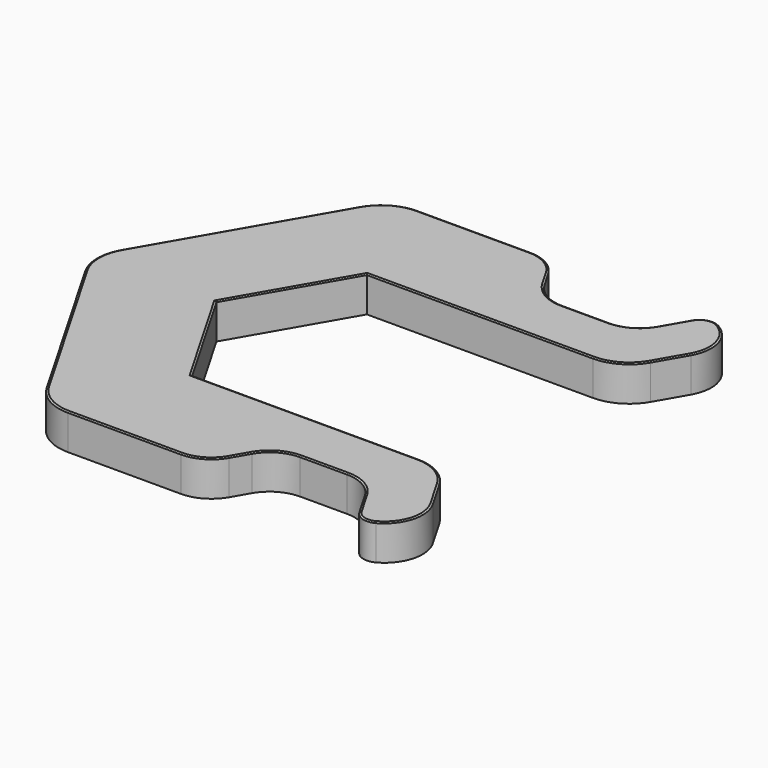
from build123d import *

# Parameters (mm, degrees)
F1_DEPTH      = 4
F2_R          = 5
F3_T1_DEPTH   = 4
F3_T3_DEPTH   = 4
F3_T5_DEPTH   = 40.2941740367
F3_T7_DEPTH   = 16.124355653
F4_R          = 1.75
F6_R          = 5
F7_T1_DEPTH   = 21.9393102292
F7_T3_DEPTH   = 21.9393102292
F7_T5_DEPTH   = 12.4011904446
F7_T7_DEPTH   = 2.0784609691
F7_T9_DEPTH   = 2.0784609691
F7_T11_DEPTH  = 5.1502577388
F7_T13_DEPTH  = 3.1580886503
F7_T15_DEPTH  = 3.1580886503
F7_T17_DEPTH  = 3.7108203073
F7_T19_DEPTH  = 3.7108203073
F7_T22_ANGLE  = 60
F7_T24_ANGLE  = 60
F7_T26_ANGLE  = 60
F7_T28_ANGLE  = 60.000000004
F7_T30_ANGLE  = 60.000000004
F7_T32_ANGLE  = 60.0000000003
F7_T34_ANGLE  = 60.0000000003
F7_T36_ANGLE  = 60.0000000003
F7_T38_ANGLE  = 60.0000000003
F7_T40_ANGLE  = 88.8306171943
F7_T42_ANGLE  = 91.1693828062
F7_T44_ANGLE  = 88.8306171943
F7_T46_ANGLE  = 91.1693828062
F7_T48_ANGLE  = 60
F7_T52_DEPTH  = 25.3440273499
F7_T55_ANGLE  = 60
F7_T59_DEPTH  = 14.8923380101
F7_T65_DEPTH  = 25.3440273499
F7_T70_DEPTH  = 14.8923380101
F7_T76_DEPTH  = 14.8923380101
F7_T82_DEPTH  = 14.8923380101
F7_T86_ANGLE  = 60
F7_T88_ANGLE  = 60
F7_T90_ANGLE  = 60
F7_T92_ANGLE  = 60.000000004
F7_T94_ANGLE  = 60.000000004
F7_T96_ANGLE  = 60.0000000003
F7_T98_ANGLE  = 60.0000000003
F7_T100_ANGLE = 60.0000000003
F7_T102_ANGLE = 60.0000000003
F7_T104_ANGLE = 88.8306171943
F7_T106_ANGLE = 91.1693828062
F7_T108_ANGLE = 88.8306171943
F7_T110_ANGLE = 91.1693828062
F7_T112_ANGLE = 60
F7_T116_DEPTH = 25.3440273499
F7_T119_ANGLE = 60
F7_T123_DEPTH = 25.3440273499
F7_T129_DEPTH = 25.3440273499
F7_T133_DEPTH = 14.8923380101
F7_T140_DEPTH = 14.8923380101
F7_T144_DEPTH = 14.8923380101
F7_T151_DEPTH = 25.3440273499
F7_T155_DEPTH = 14.8923380101
F7_T162_DEPTH = 25.3440273499
F7_T166_DEPTH = 14.8923380101
F7_T173_DEPTH = 14.8923380101
F7_T177_DEPTH = 14.8923380101
F7_T184_DEPTH = 25.3440273499
F7_T188_DEPTH = 14.8923380101


# Not quite as in the source:
# - a fillet or chamfer that OpenCascade refuses, or shapes differently, is made with other operations: its cross-section is extruded or revolved along the edge and cut away or added


with BuildPart() as f1:
    # F0 (on Top) → F1 (new body)
    with BuildSketch(Plane.XY):
        Polygon((20.7846096908, -12), (6.9282032303, -12), (-6.9282032303, -12), (-13.8564064606, 0), (-27.7128129211, 0), (-13.8564064606, -24), (3.8564064606, -24), (7.3205080757, -18), (17.3205080757, -18), align=None)
        Polygon((27.7128129211, -24), (20.7846096908, -12), (17.3205080757, -18), (20.7846096908, -24), align=None)
    extrude(amount=F1_DEPTH)

    # F2
    f2_edges = [f1.edges().sort_by_distance(p)[0] for p in [
        (-13.856406, -24, 2),
        (20.78461, -12, 2),
    ]]
    fillet(f2_edges, radius=F2_R)

    # F3: fillet of radius 4.2 on 4 edges, made by hand

    # F3_s2 → F3_t1 (join)
    with BuildSketch(Plane.XY):
        with BuildLine():
            ThreePointArc((18.532943641, -20.1), (16.9956369451, -18.5626933041), (14.8956369451, -18))
            Line((14.8956369451, -18), (17.3205080757, -18))
            Line((17.3205080757, -18), (18.532943641, -20.1))
        make_face()
    extrude(amount=F3_T1_DEPTH)

    # F3_s4 → F3_t3 (join)
    with BuildSketch(Plane.XY):
        with BuildLine():
            ThreePointArc((9.7453792063, -18), (7.6453792063, -18.5626933041), (6.1080725104, -20.1))
            Line((6.1080725104, -20.1), (7.3205080757, -18))
            Line((7.3205080757, -18), (9.7453792063, -18))
        make_face()
    extrude(amount=F3_T3_DEPTH)

    # F3_s6 → F3_t5 (cut)
    with BuildSketch(Plane.XY.offset(-18.1470870184)):
        with BuildLine():
            ThreePointArc((20.7846096908, -24), (24.165134966, -21.7652526687), (24.0833955174, -17.713664655))
            Line((24.0833955174, -17.713664655), (27.7128129211, -24))
            Line((27.7128129211, -24), (20.7846096908, -24))
        make_face()
    extrude(amount=F3_T5_DEPTH, mode=Mode.SUBTRACT)

    # F3_s8 → F3_t7 (cut)
    with BuildSketch(Plane.XY.offset(-6.0621778265)):
        with BuildLine():
            ThreePointArc((5.0688420258, -21.9), (3.53153533, -23.4373066959), (1.43153533, -24))
            Line((1.43153533, -24), (3.8564064606, -24))
            Line((3.8564064606, -24), (5.0688420258, -21.9))
        make_face()
    extrude(amount=F3_T7_DEPTH, mode=Mode.SUBTRACT)

    # F4
    f4_edges = [f1.edges().sort_by_distance(p)[0] for p in [
        (20.78461, -24, 2),
    ]]
    fillet(f4_edges, radius=F4_R)

    # F5: F1 across face


with BuildPart() as f1_1:
    add(f1.part)
    add(f1.part.mirror(Plane(origin=(-20.7846096908, 0, 2), x_dir=(-1, 0, 0), z_dir=(0, 1, 0))))

    # F6
    f6_edges = [f1_1.edges().sort_by_distance(p)[0] for p in [
        (-27.712813, 0, 2),
    ]]
    fillet(f6_edges, radius=F6_R)

    # F7: chamfer of 0.2 x 0.1 on 62 edges, made by hand

    # F7_s2 → F7_t1 (cut)
    with BuildSketch(Plane(origin=(-5.4848275573, -9.5, 0), x_dir=(0, 0, 1), z_dir=(0.5, 0.8660254038, 0))):
        Polygon((3.9, -24), (4, -23.8), (4, -24), align=None)
        Polygon((0, -23.8), (0.1, -24), (0, -24), align=None)
    extrude(amount=F7_T1_DEPTH, mode=Mode.SUBTRACT)

    # F7_s4 → F7_t3 (cut)
    with BuildSketch(Plane(origin=(-5.4848275573, 9.5, 0), x_dir=(0, 0, 1), z_dir=(0.5, -0.8660254038, 0))):
        Polygon((3.9, 24), (4, 23.8), (4, 24), align=None)
        Polygon((0, 23.8), (0.1, 24), (0, 24), align=None)
    extrude(amount=F7_T3_DEPTH, mode=Mode.SUBTRACT)

    # F7_s6 → F7_t5 (cut)
    with BuildSketch(Plane.YZ.offset(-10.9696551146)):
        Polygon((24, 3.9), (23.8, 4), (24, 4), align=None)
        Polygon((-24, 3.9), (-23.8, 4), (-24, 4), align=None)
        Polygon((-23.8, 0), (-24, 0.1), (-24, 0), align=None)
        Polygon((23.8, 0), (24, 0.1), (24, 0), align=None)
    extrude(amount=F7_T5_DEPTH, mode=Mode.SUBTRACT)

    # F7_s8 → F7_t7 (cut)
    with BuildSketch(Plane(origin=(-8.215767665, 14.2301270189, 0), x_dir=(0, 0, 1), z_dir=(0.5, -0.8660254038, 0))):
        Polygon((3.9, -15.3397459622), (4, -15.1397459622), (4, -15.3397459622), align=None)
        Polygon((0, -15.1397459622), (0.1, -15.3397459622), (0, -15.3397459622), align=None)
    extrude(amount=F7_T7_DEPTH, mode=Mode.SUBTRACT)

    # F7_s10 → F7_t9 (cut)
    with BuildSketch(Plane(origin=(-8.215767665, -14.2301270189, 0), x_dir=(0, 0, 1), z_dir=(0.5, 0.8660254038, 0))):
        Polygon((3.9, 15.3397459622), (4, 15.1397459622), (4, 15.3397459622), align=None)
        Polygon((0, 15.1397459622), (0.1, 15.3397459622), (0, 15.3397459622), align=None)
    extrude(amount=F7_T9_DEPTH, mode=Mode.SUBTRACT)

    # F7_s12 → F7_t11 (cut)
    with BuildSketch(Plane.YZ.offset(9.7453792063)):
        Polygon((18, 3.9), (17.8, 4), (18, 4), align=None)
        Polygon((-18, 3.9), (-17.8, 4), (-18, 4), align=None)
        Polygon((17.8, 0), (18, 0.1), (18, 0), align=None)
        Polygon((-17.8, 0), (-18, 0.1), (-18, 0), align=None)
    extrude(amount=F7_T11_DEPTH, mode=Mode.SUBTRACT)

    # F7_s14 → F7_t13 (cut)
    with BuildSketch(Plane(origin=(13.3367912183, 23.1, 0), x_dir=(0, 0, 1), z_dir=(0.5, 0.8660254038, 0))):
        Polygon((3.9, 6), (4, 6.2), (4, 6), align=None)
        Polygon((0, 6.2), (0.1, 6), (0, 6), align=None)
    extrude(amount=F7_T13_DEPTH, mode=Mode.SUBTRACT)

    # F7_s16 → F7_t15 (cut)
    with BuildSketch(Plane(origin=(13.3367912183, -23.1, 0), x_dir=(0, 0, 1), z_dir=(0.5, -0.8660254038, 0))):
        Polygon((3.9, -6), (4, -6.2), (4, -6), align=None)
        Polygon((0, -6.2), (0.1, -6), (0, -6), align=None)
    extrude(amount=F7_T15_DEPTH, mode=Mode.SUBTRACT)

    # F7_s18 → F7_t17 (cut)
    with BuildSketch(Plane(origin=(13.691090672, 23.713664655, 0), x_dir=(0, 0, 1), z_dir=(-0.5, -0.8660254038, 0))):
        Polygon((3.9, -12), (4, -11.8), (4, -12), align=None)
        Polygon((0, -11.8), (0.1, -12), (0, -12), align=None)
    extrude(amount=F7_T17_DEPTH, mode=Mode.SUBTRACT)

    # F7_s20 → F7_t19 (cut)
    with BuildSketch(Plane(origin=(13.691090672, -23.713664655, 0), x_dir=(0, 0, 1), z_dir=(-0.5, 0.8660254038, 0))):
        Polygon((3.9, 12), (4, 11.8), (4, 12), align=None)
        Polygon((0, 11.8), (0.1, 12), (0, 12), align=None)
    extrude(amount=F7_T19_DEPTH, mode=Mode.SUBTRACT)

    # F7_s21 → F7_t22 (revolve, cut)
    with BuildSketch(Plane(origin=(-5.4848275573, 9.5, 0), x_dir=(0, 0, 1), z_dir=(0.5, -0.8660254038, 0))):
        Polygon((3.9, 24), (4, 23.8), (4, 24), align=None)
    revolve(axis=Axis((-21.9393102292, 0, 4), (0, 0, -1)), revolution_arc=F7_T22_ANGLE, mode=Mode.SUBTRACT)

    # F7_s23 → F7_t24 (revolve, cut)
    with BuildSketch(Plane(origin=(5.4848275573, 9.5, 0), x_dir=(0, 0, 1), z_dir=(-0.5, -0.8660254038, 0))):
        Polygon((3.9, 24), (4, 23.8), (4, 24), align=None)
    revolve(axis=Axis((-10.9696551146, 19, 4), (0, 0, -1)), revolution_arc=F7_T24_ANGLE, mode=Mode.SUBTRACT)

    # F7_s25 → F7_t26 (revolve, cut)
    with BuildSketch(Plane(origin=(5.4848275573, -9.5, 0), x_dir=(0, 0, 1), z_dir=(-0.5, 0.8660254038, 0))):
        Polygon((3.9, -24), (4, -23.8), (4, -24), align=None)
    revolve(axis=Axis((-10.9696551146, -19, 4), (0, 0, 1)), revolution_arc=F7_T26_ANGLE, mode=Mode.SUBTRACT)

    # F7_s27 → F7_t28 (revolve, cut)
    with BuildSketch(Plane(origin=(-8.2157676647, 14.2301270199, 0), x_dir=(0, 0, 1), z_dir=(0.5, -0.8660254038, 0))):
        Polygon((3.9, -15.3397459614), (4, -15.1397459614), (4, -15.3397459614), align=None)
    revolve(axis=Axis((1.4315353301, 19.8000000003, 4), (0, 0, 1)), revolution_arc=F7_T28_ANGLE, mode=Mode.SUBTRACT)

    # F7_s29 → F7_t30 (revolve, cut)
    with BuildSketch(Plane(origin=(-8.2157676647, -14.2301270199, 0), x_dir=(0, 0, 1), z_dir=(0.5, 0.8660254038, 0))):
        Polygon((3.9, 15.3397459614), (4, 15.1397459614), (4, 15.3397459614), align=None)
    revolve(axis=Axis((1.4315353301, -19.8000000003, 4), (0, 0, -1)), revolution_arc=F7_T30_ANGLE, mode=Mode.SUBTRACT)

    # F7_s31 → F7_t32 (revolve, cut)
    with BuildSketch(Plane.YZ.offset(9.7453792063)):
        Polygon((18, 3.9), (17.8, 4), (18, 4), align=None)
    revolve(axis=Axis((9.7453792063, 22.2, 4), (0, 0, -1)), revolution_arc=F7_T32_ANGLE, mode=Mode.SUBTRACT)

    # F7_s33 → F7_t34 (revolve, cut)
    with BuildSketch(Plane.YZ.offset(9.7453792063)):
        Polygon((-18, 3.9), (-17.8, 4), (-18, 4), align=None)
    revolve(axis=Axis((9.7453792063, -22.2, 4), (0, 0, 1)), revolution_arc=F7_T34_ANGLE, mode=Mode.SUBTRACT)

    # F7_s35 → F7_t36 (revolve, cut)
    with BuildSketch(Plane(origin=(13.3367912182, 23.1, 0), x_dir=(0, 0, 1), z_dir=(0.5, 0.8660254038, 0))):
        Polygon((3.9, 6.0000000001), (4, 6.2000000001), (4, 6.0000000001), align=None)
    revolve(axis=Axis((14.8956369451, 22.2, 4), (0, 0, -1)), revolution_arc=F7_T36_ANGLE, mode=Mode.SUBTRACT)

    # F7_s37 → F7_t38 (revolve, cut)
    with BuildSketch(Plane(origin=(13.3367912182, -23.1, 0), x_dir=(0, 0, 1), z_dir=(0.5, -0.8660254038, 0))):
        Polygon((3.9, -6.0000000001), (4, -6.2000000001), (4, -6.0000000001), align=None)
    revolve(axis=Axis((14.8956369451, -22.2, 4), (0, 0, 1)), revolution_arc=F7_T38_ANGLE, mode=Mode.SUBTRACT)

    # F7_s39 → F7_t40 (revolve, cut)
    with BuildSketch(Plane(origin=(7.3213137927, -4.0300225261, 0), x_dir=(0, 0, 1), z_dir=(0.8760491198, -0.482221878, 0))):
        Polygon((3.9, -31.4172948315), (4, -31.2172948315), (4, -31.4172948315), align=None)
    revolve(axis=Axis((21.6275324227, 21.9599849985, 4), (0, 0, 1)), revolution_arc=F7_T40_ANGLE, mode=Mode.SUBTRACT)

    # F7_s41 → F7_t42 (revolve, cut)
    with BuildSketch(Plane(origin=(13.6910906723, 23.7136646549, 0), x_dir=(0, 0, 1), z_dir=(-0.5, -0.8660254038, 0))):
        Polygon((3.9, -11.9999999997), (4, -11.7999999997), (4, -11.9999999997), align=None)
    revolve(axis=Axis((20.4460888216, 19.813664655, 4), (0, 0, 1)), revolution_arc=F7_T42_ANGLE, mode=Mode.SUBTRACT)

    # F7_s43 → F7_t44 (revolve, cut)
    with BuildSketch(Plane(origin=(7.3213137927, 4.0300225261, 0), x_dir=(0, 0, 1), z_dir=(0.8760491198, 0.482221878, 0))):
        Polygon((3.9, 31.4172948315), (4, 31.2172948315), (4, 31.4172948315), align=None)
    revolve(axis=Axis((21.6275324227, -21.9599849985, 4), (0, 0, -1)), revolution_arc=F7_T44_ANGLE, mode=Mode.SUBTRACT)

    # F7_s45 → F7_t46 (revolve, cut)
    with BuildSketch(Plane(origin=(13.6910906723, -23.7136646549, 0), x_dir=(0, 0, 1), z_dir=(-0.5, 0.8660254038, 0))):
        Polygon((3.9, 11.9999999997), (4, 11.7999999997), (4, 11.9999999997), align=None)
    revolve(axis=Axis((20.4460888216, -19.813664655, 4), (0, 0, -1)), revolution_arc=F7_T46_ANGLE, mode=Mode.SUBTRACT)

    # F7_s47 → F7_t48 (revolve, cut)
    with BuildSketch(Plane.YZ.offset(17.8978583449)):
        Polygon((12, 3.9), (12.2, 4), (12, 4), align=None)
    revolve(axis=Axis((17.8978583449, 17, 4), (0, 0, 1)), revolution_arc=F7_T48_ANGLE, mode=Mode.SUBTRACT)


with BuildPart() as f7_tool50:
    # F7_s51 → F7_t52 (new body)
    with BuildSketch(Plane.YZ.offset(17.8978583449)):
        Polygon((12, 3.9), (12.2, 4), (12, 4), align=None)
    extrude(amount=-F7_T52_DEPTH)

    split(bisect_by=Plane(origin=(-10.3923048454, 6, 0), x_dir=(0, 0, 1), z_dir=(0.8660254038, -0.5, 0)), keep=Keep.TOP)


with BuildPart() as f1_2:
    add(f1_1.part)

    # F7_t49: cut F7_tool50
    add(f7_tool50.part, mode=Mode.SUBTRACT)

    # F7_s54 → F7_t55 (revolve, cut)
    with BuildSketch(Plane.YZ.offset(17.8978583449)):
        Polygon((-12, 3.9), (-12.2, 4), (-12, 4), align=None)
    revolve(axis=Axis((17.8978583449, -17, 4), (0, 0, -1)), revolution_arc=F7_T55_ANGLE, mode=Mode.SUBTRACT)


with BuildPart() as f7_tool57:
    # F7_s58 → F7_t59 (new body)
    with BuildSketch(Plane(origin=(3.7230845025, 6.4485715192, 0), x_dir=(0, 0, 1), z_dir=(-0.5, -0.8660254038, 0))):
        Polygon((3.9, 12), (4, 12.2), (4, 12), align=None)
    extrude(amount=F7_T59_DEPTH)

    split(bisect_by=Plane.XZ.offset(-12), keep=Keep.TOP)

    split(bisect_by=Plane(origin=(-10.3923048454, -6, 0), x_dir=(0, 0, 1), z_dir=(0.8660254038, 0.5, 0)), keep=Keep.TOP)


with BuildPart() as f1_3:
    add(f1_2.part)

    # F7_t56: cut F7_tool57
    add(f7_tool57.part, mode=Mode.SUBTRACT)


with BuildPart() as f7_tool63:
    # F7_s64 → F7_t65 (new body)
    with BuildSketch(Plane.YZ.offset(17.8978583449)):
        Polygon((-12, 3.9), (-12.2, 4), (-12, 4), align=None)
    extrude(amount=-F7_T65_DEPTH)

    split(bisect_by=Plane(origin=(-10.3923048454, -6, 0), x_dir=(0, 0, 1), z_dir=(0.8660254038, 0.5, 0)), keep=Keep.TOP)


with BuildPart() as f1_4:
    add(f1_3.part)

    # F7_t62: cut F7_tool63
    add(f7_tool63.part, mode=Mode.SUBTRACT)


with BuildPart() as f7_tool68:
    # F7_s69 → F7_t70 (new body)
    with BuildSketch(Plane(origin=(3.7230845025, -6.4485715192, 0), x_dir=(0, 0, 1), z_dir=(-0.5, 0.8660254038, 0))):
        Polygon((3.9, -12), (4, -12.2), (4, -12), align=None)
    extrude(amount=F7_T70_DEPTH)

    split(bisect_by=Plane(origin=(-10.3923048454, 6, 0), x_dir=(0, 0, 1), z_dir=(0.8660254038, -0.5, 0)), keep=Keep.TOP)

    split(bisect_by=Plane.XZ.offset(12), keep=Keep.BOTTOM)


with BuildPart() as f1_5:
    add(f1_4.part)

    # F7_t67: cut F7_tool68
    add(f7_tool68.part, mode=Mode.SUBTRACT)


with BuildPart() as f7_tool74:
    # F7_s75 → F7_t76 (new body)
    with BuildSketch(Plane(origin=(3.7230845025, -6.4485715192, 0), x_dir=(0, 0, 1), z_dir=(-0.5, 0.8660254038, 0))):
        Polygon((0, -12.2), (0.1, -12), (0, -12), align=None)
    extrude(amount=F7_T76_DEPTH)

    split(bisect_by=Plane(origin=(-10.3923048454, 6, 0), x_dir=(0, 0, 1), z_dir=(0.8660254038, -0.5, 0)), keep=Keep.TOP)

    split(bisect_by=Plane.XZ.offset(12), keep=Keep.BOTTOM)


with BuildPart() as f1_6:
    add(f1_5.part)

    # F7_t73: cut F7_tool74
    add(f7_tool74.part, mode=Mode.SUBTRACT)


with BuildPart() as f7_tool80:
    # F7_s81 → F7_t82 (new body)
    with BuildSketch(Plane(origin=(3.7230845025, 6.4485715192, 0), x_dir=(0, 0, 1), z_dir=(-0.5, -0.8660254038, 0))):
        Polygon((0, 12.2), (0.1, 12), (0, 12), align=None)
    extrude(amount=F7_T82_DEPTH)

    split(bisect_by=Plane.XZ.offset(-12), keep=Keep.TOP)

    split(bisect_by=Plane(origin=(-10.3923048454, -6, 0), x_dir=(0, 0, 1), z_dir=(0.8660254038, 0.5, 0)), keep=Keep.TOP)


with BuildPart() as f1_7:
    add(f1_6.part)

    # F7_t79: cut F7_tool80
    add(f7_tool80.part, mode=Mode.SUBTRACT)

    # F7_s85 → F7_t86 (revolve, cut)
    with BuildSketch(Plane(origin=(-5.4848275573, 9.5, 0), x_dir=(0, 0, 1), z_dir=(0.5, -0.8660254038, 0))):
        Polygon((0, 23.8), (0.1, 24), (0, 24), align=None)
    revolve(axis=Axis((-21.9393102292, 0, 0), (0, 0, -1)), revolution_arc=F7_T86_ANGLE, mode=Mode.SUBTRACT)

    # F7_s87 → F7_t88 (revolve, cut)
    with BuildSketch(Plane(origin=(5.4848275573, 9.5, 0), x_dir=(0, 0, 1), z_dir=(-0.5, -0.8660254038, 0))):
        Polygon((0, 23.8), (0.1, 24), (0, 24), align=None)
    revolve(axis=Axis((-10.9696551146, 19, 0), (0, 0, -1)), revolution_arc=F7_T88_ANGLE, mode=Mode.SUBTRACT)

    # F7_s89 → F7_t90 (revolve, cut)
    with BuildSketch(Plane(origin=(5.4848275573, -9.5, 0), x_dir=(0, 0, 1), z_dir=(-0.5, 0.8660254038, 0))):
        Polygon((0, -23.8), (0.1, -24), (0, -24), align=None)
    revolve(axis=Axis((-10.9696551146, -19, 0), (0, 0, 1)), revolution_arc=F7_T90_ANGLE, mode=Mode.SUBTRACT)

    # F7_s91 → F7_t92 (revolve, cut)
    with BuildSketch(Plane(origin=(-8.2157676647, 14.2301270199, 0), x_dir=(0, 0, 1), z_dir=(0.5, -0.8660254038, 0))):
        Polygon((0, -15.1397459614), (0.1, -15.3397459614), (0, -15.3397459614), align=None)
    revolve(axis=Axis((1.4315353301, 19.8000000003, 0), (0, 0, 1)), revolution_arc=F7_T92_ANGLE, mode=Mode.SUBTRACT)

    # F7_s93 → F7_t94 (revolve, cut)
    with BuildSketch(Plane(origin=(-8.2157676647, -14.2301270199, 0), x_dir=(0, 0, 1), z_dir=(0.5, 0.8660254038, 0))):
        Polygon((0, 15.1397459614), (0.1, 15.3397459614), (0, 15.3397459614), align=None)
    revolve(axis=Axis((1.4315353301, -19.8000000003, 0), (0, 0, -1)), revolution_arc=F7_T94_ANGLE, mode=Mode.SUBTRACT)

    # F7_s95 → F7_t96 (revolve, cut)
    with BuildSketch(Plane.YZ.offset(9.7453792063)):
        Polygon((17.8, 0), (18, 0.1), (18, 0), align=None)
    revolve(axis=Axis((9.7453792063, 22.2, 0), (0, 0, -1)), revolution_arc=F7_T96_ANGLE, mode=Mode.SUBTRACT)

    # F7_s97 → F7_t98 (revolve, cut)
    with BuildSketch(Plane.YZ.offset(9.7453792063)):
        Polygon((-17.8, 0), (-18, 0.1), (-18, 0), align=None)
    revolve(axis=Axis((9.7453792063, -22.2, 0), (0, 0, 1)), revolution_arc=F7_T98_ANGLE, mode=Mode.SUBTRACT)

    # F7_s99 → F7_t100 (revolve, cut)
    with BuildSketch(Plane(origin=(13.3367912182, 23.1, 0), x_dir=(0, 0, 1), z_dir=(0.5, 0.8660254038, 0))):
        Polygon((0, 6.2000000001), (0.1, 6.0000000001), (0, 6.0000000001), align=None)
    revolve(axis=Axis((14.8956369451, 22.2, 0), (0, 0, -1)), revolution_arc=F7_T100_ANGLE, mode=Mode.SUBTRACT)

    # F7_s101 → F7_t102 (revolve, cut)
    with BuildSketch(Plane(origin=(13.3367912182, -23.1, 0), x_dir=(0, 0, 1), z_dir=(0.5, -0.8660254038, 0))):
        Polygon((0, -6.2000000001), (0.1, -6.0000000001), (0, -6.0000000001), align=None)
    revolve(axis=Axis((14.8956369451, -22.2, 0), (0, 0, 1)), revolution_arc=F7_T102_ANGLE, mode=Mode.SUBTRACT)

    # F7_s103 → F7_t104 (revolve, cut)
    with BuildSketch(Plane(origin=(7.3213137927, -4.0300225261, 0), x_dir=(0, 0, 1), z_dir=(0.8760491198, -0.482221878, 0))):
        Polygon((0, -31.2172948315), (0.1, -31.4172948315), (0, -31.4172948315), align=None)
    revolve(axis=Axis((21.6275324227, 21.9599849985, 0), (0, 0, 1)), revolution_arc=F7_T104_ANGLE, mode=Mode.SUBTRACT)

    # F7_s105 → F7_t106 (revolve, cut)
    with BuildSketch(Plane(origin=(13.6910906723, 23.7136646549, 0), x_dir=(0, 0, 1), z_dir=(-0.5, -0.8660254038, 0))):
        Polygon((0, -11.7999999997), (0.1, -11.9999999997), (0, -11.9999999997), align=None)
    revolve(axis=Axis((20.4460888216, 19.813664655, 0), (0, 0, 1)), revolution_arc=F7_T106_ANGLE, mode=Mode.SUBTRACT)

    # F7_s107 → F7_t108 (revolve, cut)
    with BuildSketch(Plane(origin=(7.3213137927, 4.0300225261, 0), x_dir=(0, 0, 1), z_dir=(0.8760491198, 0.482221878, 0))):
        Polygon((0, 31.2172948315), (0.1, 31.4172948315), (0, 31.4172948315), align=None)
    revolve(axis=Axis((21.6275324227, -21.9599849985, 0), (0, 0, -1)), revolution_arc=F7_T108_ANGLE, mode=Mode.SUBTRACT)

    # F7_s109 → F7_t110 (revolve, cut)
    with BuildSketch(Plane(origin=(13.6910906723, -23.7136646549, 0), x_dir=(0, 0, 1), z_dir=(-0.5, 0.8660254038, 0))):
        Polygon((0, 11.7999999997), (0.1, 11.9999999997), (0, 11.9999999997), align=None)
    revolve(axis=Axis((20.4460888216, -19.813664655, 0), (0, 0, -1)), revolution_arc=F7_T110_ANGLE, mode=Mode.SUBTRACT)

    # F7_s111 → F7_t112 (revolve, cut)
    with BuildSketch(Plane.YZ.offset(17.8978583449)):
        Polygon((12.2, 0), (12, 0.1), (12, 0), align=None)
    revolve(axis=Axis((17.8978583449, 17, 0), (0, 0, 1)), revolution_arc=F7_T112_ANGLE, mode=Mode.SUBTRACT)


with BuildPart() as f7_tool114:
    # F7_s115 → F7_t116 (new body)
    with BuildSketch(Plane.YZ.offset(17.8978583449)):
        Polygon((12.2, 0), (12, 0.1), (12, 0), align=None)
    extrude(amount=-F7_T116_DEPTH)

    split(bisect_by=Plane(origin=(-10.3923048454, 6, 0), x_dir=(0, 0, 1), z_dir=(0.8660254038, -0.5, 0)), keep=Keep.TOP)


with BuildPart() as f1_8:
    add(f1_7.part)

    # F7_t113: cut F7_tool114
    add(f7_tool114.part, mode=Mode.SUBTRACT)

    # F7_s118 → F7_t119 (revolve, cut)
    with BuildSketch(Plane.YZ.offset(17.8978583449)):
        Polygon((-12.2, 0), (-12, 0.1), (-12, 0), align=None)
    revolve(axis=Axis((17.8978583449, -17, 0), (0, 0, -1)), revolution_arc=F7_T119_ANGLE, mode=Mode.SUBTRACT)


with BuildPart() as f7_tool121:
    # F7_s122 → F7_t123 (new body)
    with BuildSketch(Plane.YZ.offset(17.8978583449)):
        Polygon((-12.2, 0), (-12, 0.1), (-12, 0), align=None)
    extrude(amount=-F7_T123_DEPTH)

    split(bisect_by=Plane(origin=(-10.3923048454, -6, 0), x_dir=(0, 0, 1), z_dir=(0.8660254038, 0.5, 0)), keep=Keep.TOP)


with BuildPart() as f1_9:
    add(f1_8.part)

    # F7_t120: cut F7_tool121
    add(f7_tool121.part, mode=Mode.SUBTRACT)


with BuildPart() as f7_tool127:
    # F7_s128 → F7_t129 (new body)
    with BuildSketch(Plane.YZ.offset(17.8978583449)):
        Polygon((12, 3.9), (12.2, 4), (12, 4), align=None)
    extrude(amount=-F7_T129_DEPTH)

    split(bisect_by=Plane(origin=(-10.3923048454, 6, 0), x_dir=(0, 0, 1), z_dir=(-0.8660254038, 0.5, 0)), keep=Keep.TOP)


with BuildPart() as f7_tool131:
    # F7_s132 → F7_t133 (new body)
    with BuildSketch(Plane(origin=(3.7230845025, 6.4485715192, 0), x_dir=(0, 0, 1), z_dir=(-0.5, -0.8660254038, 0))):
        Polygon((3.9, 12), (4, 12.2), (4, 12), align=None)
    extrude(amount=F7_T133_DEPTH)

    split(bisect_by=Plane.XZ.offset(-12), keep=Keep.BOTTOM)


with BuildPart() as f7_tool127_1:
    add(f7_tool127.part)

    # F7_t135: intersect F7_tool131
    add(f7_tool131.part, mode=Mode.INTERSECT)


with BuildPart() as f1_10:
    add(f1_9.part)

    # F7_t125: cut F7_tool127
    add(f7_tool127_1.part, mode=Mode.SUBTRACT)


with BuildPart() as f7_tool138:
    # F7_s139 → F7_t140 (new body)
    with BuildSketch(Plane(origin=(3.7230845025, 6.4485715192, 0), x_dir=(0, 0, 1), z_dir=(-0.5, -0.8660254038, 0))):
        Polygon((3.9, 12), (4, 12.2), (4, 12), align=None)
    extrude(amount=F7_T140_DEPTH)

    split(bisect_by=Plane(origin=(-10.3923048454, -6, 0), x_dir=(0, 0, 1), z_dir=(-0.8660254038, -0.5, 0)), keep=Keep.TOP)


with BuildPart() as f7_tool142:
    # F7_s143 → F7_t144 (new body)
    with BuildSketch(Plane(origin=(3.7230845025, -6.4485715192, 0), x_dir=(0, 0, 1), z_dir=(-0.5, 0.8660254038, 0))):
        Polygon((3.9, -12), (4, -12.2), (4, -12), align=None)
    extrude(amount=F7_T144_DEPTH)

    split(bisect_by=Plane(origin=(-10.3923048454, 6, 0), x_dir=(0, 0, 1), z_dir=(-0.8660254038, 0.5, 0)), keep=Keep.TOP)


with BuildPart() as f7_tool138_1:
    add(f7_tool138.part)

    # F7_t146: intersect F7_tool142
    add(f7_tool142.part, mode=Mode.INTERSECT)


with BuildPart() as f1_11:
    add(f1_10.part)

    # F7_t136: cut F7_tool138
    add(f7_tool138_1.part, mode=Mode.SUBTRACT)


with BuildPart() as f7_tool149:
    # F7_s150 → F7_t151 (new body)
    with BuildSketch(Plane.YZ.offset(17.8978583449)):
        Polygon((-12, 3.9), (-12.2, 4), (-12, 4), align=None)
    extrude(amount=-F7_T151_DEPTH)

    split(bisect_by=Plane(origin=(-10.3923048454, -6, 0), x_dir=(0, 0, 1), z_dir=(-0.8660254038, -0.5, 0)), keep=Keep.TOP)


with BuildPart() as f7_tool153:
    # F7_s154 → F7_t155 (new body)
    with BuildSketch(Plane(origin=(3.7230845025, -6.4485715192, 0), x_dir=(0, 0, 1), z_dir=(-0.5, 0.8660254038, 0))):
        Polygon((3.9, -12), (4, -12.2), (4, -12), align=None)
    extrude(amount=F7_T155_DEPTH)

    split(bisect_by=Plane.XZ.offset(12), keep=Keep.TOP)


with BuildPart() as f7_tool149_1:
    add(f7_tool149.part)

    # F7_t157: intersect F7_tool153
    add(f7_tool153.part, mode=Mode.INTERSECT)


with BuildPart() as f1_12:
    add(f1_11.part)

    # F7_t147: cut F7_tool149
    add(f7_tool149_1.part, mode=Mode.SUBTRACT)


with BuildPart() as f7_tool160:
    # F7_s161 → F7_t162 (new body)
    with BuildSketch(Plane.YZ.offset(17.8978583449)):
        Polygon((-12.2, 0), (-12, 0.1), (-12, 0), align=None)
    extrude(amount=-F7_T162_DEPTH)

    split(bisect_by=Plane(origin=(-10.3923048454, -6, 0), x_dir=(0, 0, 1), z_dir=(-0.8660254038, -0.5, 0)), keep=Keep.TOP)


with BuildPart() as f7_tool164:
    # F7_s165 → F7_t166 (new body)
    with BuildSketch(Plane(origin=(3.7230845025, -6.4485715192, 0), x_dir=(0, 0, 1), z_dir=(-0.5, 0.8660254038, 0))):
        Polygon((0, -12.2), (0.1, -12), (0, -12), align=None)
    extrude(amount=F7_T166_DEPTH)

    split(bisect_by=Plane.XZ.offset(12), keep=Keep.TOP)


with BuildPart() as f7_tool160_1:
    add(f7_tool160.part)

    # F7_t168: intersect F7_tool164
    add(f7_tool164.part, mode=Mode.INTERSECT)


with BuildPart() as f1_13:
    add(f1_12.part)

    # F7_t158: cut F7_tool160
    add(f7_tool160_1.part, mode=Mode.SUBTRACT)


with BuildPart() as f7_tool171:
    # F7_s172 → F7_t173 (new body)
    with BuildSketch(Plane(origin=(3.7230845025, 6.4485715192, 0), x_dir=(0, 0, 1), z_dir=(-0.5, -0.8660254038, 0))):
        Polygon((0, 12.2), (0.1, 12), (0, 12), align=None)
    extrude(amount=F7_T173_DEPTH)

    split(bisect_by=Plane(origin=(-10.3923048454, -6, 0), x_dir=(0, 0, 1), z_dir=(-0.8660254038, -0.5, 0)), keep=Keep.TOP)


with BuildPart() as f7_tool175:
    # F7_s176 → F7_t177 (new body)
    with BuildSketch(Plane(origin=(3.7230845025, -6.4485715192, 0), x_dir=(0, 0, 1), z_dir=(-0.5, 0.8660254038, 0))):
        Polygon((0, -12.2), (0.1, -12), (0, -12), align=None)
    extrude(amount=F7_T177_DEPTH)

    split(bisect_by=Plane(origin=(-10.3923048454, 6, 0), x_dir=(0, 0, 1), z_dir=(-0.8660254038, 0.5, 0)), keep=Keep.TOP)


with BuildPart() as f7_tool171_1:
    add(f7_tool171.part)

    # F7_t179: intersect F7_tool175
    add(f7_tool175.part, mode=Mode.INTERSECT)


with BuildPart() as f1_14:
    add(f1_13.part)

    # F7_t169: cut F7_tool171
    add(f7_tool171_1.part, mode=Mode.SUBTRACT)


with BuildPart() as f7_tool182:
    # F7_s183 → F7_t184 (new body)
    with BuildSketch(Plane.YZ.offset(17.8978583449)):
        Polygon((12.2, 0), (12, 0.1), (12, 0), align=None)
    extrude(amount=-F7_T184_DEPTH)

    split(bisect_by=Plane(origin=(-10.3923048454, 6, 0), x_dir=(0, 0, 1), z_dir=(-0.8660254038, 0.5, 0)), keep=Keep.TOP)


with BuildPart() as f7_tool186:
    # F7_s187 → F7_t188 (new body)
    with BuildSketch(Plane(origin=(3.7230845025, 6.4485715192, 0), x_dir=(0, 0, 1), z_dir=(-0.5, -0.8660254038, 0))):
        Polygon((0, 12.2), (0.1, 12), (0, 12), align=None)
    extrude(amount=F7_T188_DEPTH)

    split(bisect_by=Plane.XZ.offset(-12), keep=Keep.BOTTOM)


with BuildPart() as f7_tool182_1:
    add(f7_tool182.part)

    # F7_t190: intersect F7_tool186
    add(f7_tool186.part, mode=Mode.INTERSECT)


with BuildPart() as f1_15:
    add(f1_14.part)

    # F7_t180: cut F7_tool182
    add(f7_tool182_1.part, mode=Mode.SUBTRACT)


solid = f1_15.part
